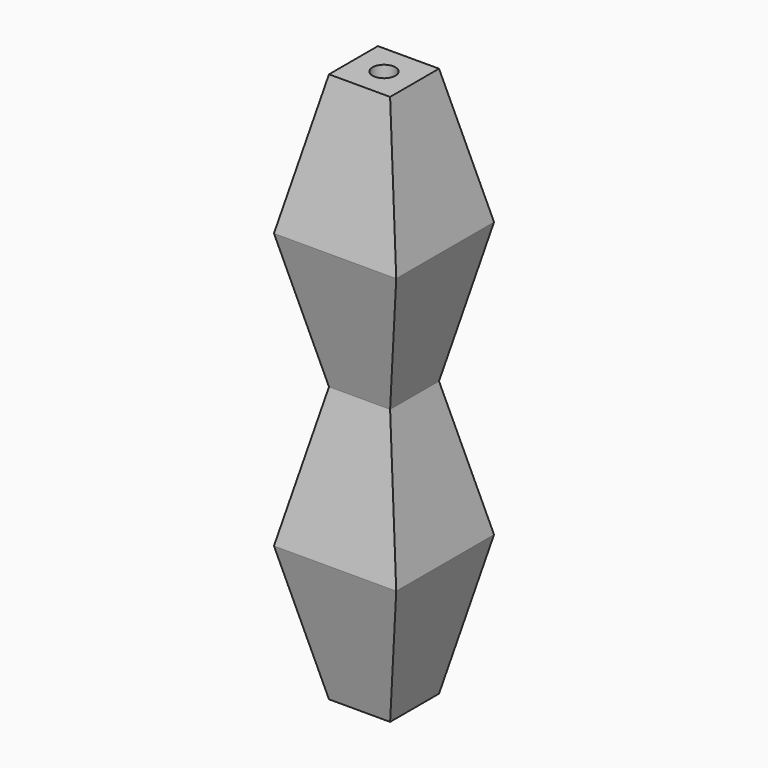
from build123d import *

# Parameters (mm, degrees)
F0_W          = 101.6
F0_H          = 101.6
F1_DEPTH      = 457.2
F3_DEPTH      = 50.801
F3_DEPTH_BACK = 50.801
F5_DEPTH      = 50.801
F5_DEPTH_BACK = 50.801
F6_R          = 9.525
F7_DEPTH      = 457.201
F7_DEPTH_BACK = 708


# Not quite as in the source:
# - an extrude ends at something that could not be found from the text; its depth is read off the source's solid


with BuildPart() as f1:
    # F0 (on Top) → F1 (new body)
    with BuildSketch(Plane.XY):
        Rectangle(F0_W, F0_H)
    extrude(amount=F1_DEPTH)

    # F2 (on Front) → F3 (cut, two sides)
    with BuildSketch(Plane.XZ) as f3_sk:
        Polygon((-76.2, 0), (-50.8, 0), (-25.4, 0), (-50.8, 114.3), (-25.4, 228.6), (-50.8, 342.9), (-25.4, 457.2), (-50.8, 457.2), (-76.2, 457.2), align=None)
        Polygon((76.2, 457.2), (50.8, 457.2), (25.4, 457.2), (50.8, 342.9), (25.4, 228.6), (50.8, 114.3), (25.4, 0), (50.8, 0), (76.2, 0), align=None)
    extrude(amount=-F3_DEPTH, mode=Mode.SUBTRACT)
    extrude(f3_sk.sketch, amount=F3_DEPTH_BACK, mode=Mode.SUBTRACT)

    # F4 (on Right) → F5 (cut, two sides)
    with BuildSketch(Plane.YZ) as f5_sk:
        Polygon((76.2, 457.2), (50.8, 457.2), (25.4, 457.2), (50.8, 342.9), (25.4, 228.6), (50.8, 114.3), (25.4, 0), (50.8, 0), (76.2, 0), align=None)
        Polygon((-25.4, 457.2), (-50.8, 457.2), (-76.2, 457.2), (-76.2, 0), (-50.8, 0), (-25.4, 0), (-50.8, 114.3), (-25.4, 228.6), (-50.8, 342.9), align=None)
    extrude(amount=-F5_DEPTH, mode=Mode.SUBTRACT)
    extrude(f5_sk.sketch, amount=F5_DEPTH_BACK, mode=Mode.SUBTRACT)

    # F6 (on Top) → F7 (cut, two sides)
    with BuildSketch(Plane.XY) as f7_sk:
        Circle(F6_R)
    extrude(amount=F7_DEPTH, mode=Mode.SUBTRACT)
    extrude(f7_sk.sketch, amount=-F7_DEPTH_BACK, mode=Mode.SUBTRACT)


solid = f1.part
